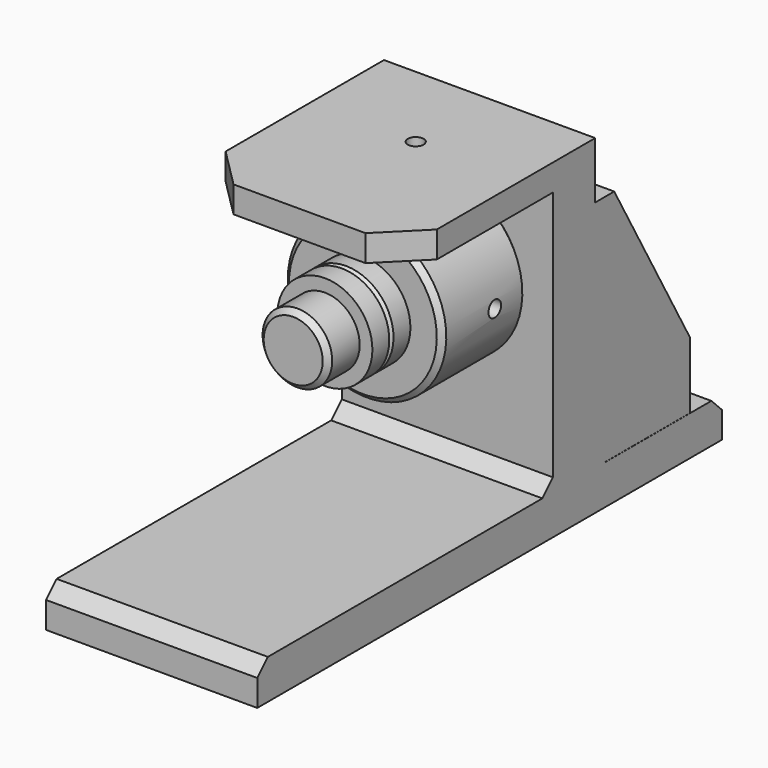
from build123d import *

# Parameters (mm, degrees)
F2_SIZE         = 2
F4_COPIES_COUNT = 4
F6_W            = 2
F6_H            = 10
F8_W            = 80
F8_H            = 90
F8_R            = 5
F9_DEPTH        = 10
F10_SIZE        = 15
F12_W           = 80
F12_H           = 100
F13_DEPTH       = 20
F15_DEPTH       = 80
F17_W           = 80
F17_H           = 15
F18_DEPTH       = 120
F18_DEPTH_BACK  = 100
F19_SIZE        = 5
F20_R           = 5
F21_DEPTH       = 10
F22_SIZE        = 2
F23_DEPTH       = 40
F23_DEPTH_BACK  = 40
F24_DEPTH       = 25
F24_DEPTH_BACK  = 25
F25_W           = 7
F25_H           = 20
F31_SIZE        = 2


# Not quite as in the source:
# - a pattern or mirror of a feature is missing from the dataset's text; its kind, count and spacing are read off the source's solid


with BuildPart() as f1:
    # F0 (on Right) → F1 (revolve)
    with BuildSketch(Plane.YZ):
        Polygon((-10, 18), (-10, 11), (40, 11), (40, 30), (0, 30), (0, 18), align=None)
    revolve(axis=Axis((0, 15, 0), (0, -1, 0)))

    # F2
    f2_edges = [f1.edges().sort_by_distance(p)[0] for p in [
        (0, -10, -18),
        (0, 0, -30),
        (0, 40, -30),
    ]]
    chamfer(f2_edges, length=F2_SIZE)

    # F3 (on Right) → F4 (revolve, cut)
    with BuildSketch(Plane.YZ):
        Polygon((22, 18), (25, 16.2679491924), (25, 30), (22, 30), align=None)
    f4 = revolve(axis=Axis((0, 25, 23.1339745962), (0, 0, 1)), mode=Mode.SUBTRACT)

    # F4_copies: F4 ×4 about axis
    f4_copies_axis = Axis((0, 0, 0), (0, 1, 0))
    for i in range(1, F4_COPIES_COUNT):
        add(f4.rotate(f4_copies_axis, i * 360 / F4_COPIES_COUNT), mode=Mode.SUBTRACT)


with BuildPart() as f7:
    # F6 (on Right) → F7 (revolve)
    with BuildSketch(Plane.YZ):
        with Locations((21, 41)):
            Rectangle(F6_W, F6_H)
    revolve(axis=Axis((0, 25, 40.9752885997), (0, 0, -1)))

    # F8 (on offset) → F9 (join)
    with BuildSketch(Plane.XY.offset(46)):
        with Locations((0, 15)):
            Rectangle(F8_W, F8_H)
        with Locations((0, 25)):
            Circle(F8_R, mode=Mode.SUBTRACT)
    extrude(amount=-F9_DEPTH)

    # F10
    f10_edges = [f7.edges().sort_by_distance(p)[0] for p in [
        (-40, -30, 41),
        (40, -30, 41),
    ]]
    chamfer(f10_edges, length=F10_SIZE)

    # F12 (on offset) → F13 (join)
    with BuildSketch(Plane.XZ.offset(-60)):
        with Locations((0, -14)):
            Rectangle(F12_W, F12_H)
    extrude(amount=F13_DEPTH)

    # F14 (on face) → F15 (join)
    with BuildSketch(Plane.YZ.offset(40)):
        Polygon((35, -64), (40, -64), (40, -59), align=None)
        Polygon((60, -59), (60, -64), (65, -64), align=None)
    extrude(amount=-F15_DEPTH)

    # F17 (on Front) → F18 (join, two sides)
    with BuildSketch(Plane.XZ) as f18_sk:
        with Locations((0, -71.5)):
            Rectangle(F17_W, F17_H)
    extrude(amount=-F18_DEPTH)
    extrude(f18_sk.sketch, amount=F18_DEPTH_BACK)

    # F19
    f19_edges = [f7.edges().sort_by_distance(p)[0] for p in [
        (0, 120, -64),
        (0, -100, -64),
    ]]
    chamfer(f19_edges, length=F19_SIZE)

    # F20 (on face) → F21 (join)
    with BuildSketch(Plane(origin=(0, 0, -79), x_dir=(1, 0, 0), z_dir=(0, 0, -1))):
        with Locations((0, 50)):
            Circle(F20_R)
        with Locations((0, -70)):
            Circle(F20_R)
    extrude(amount=F21_DEPTH)

    # F22
    f22_edges = [f7.edges().sort_by_distance(p)[0] for p in [
        (-5, -50, -89),
        (-5, 70, -89),
    ]]
    chamfer(f22_edges, length=F22_SIZE)

    # F16 (on Right) → F23 (join, two sides)
    with BuildSketch(Plane.YZ) as f23_sk:
        Polygon((69, 24.5257518999), (60, 24.5257518999), (60, -63.9528611181), (105, -63.9528611181), (105, -38.9528611181), align=None)
    extrude(amount=F23_DEPTH)
    extrude(f23_sk.sketch, amount=-F23_DEPTH_BACK)

    # F16 (on Right) → F24 (cut, two sides)
    with BuildSketch(Plane.YZ) as f24_sk:
        Polygon((69, 24.5257518999), (60, 24.5257518999), (60, -63.9528611181), (105, -63.9528611181), (105, -38.9528611181), align=None)
    extrude(amount=F24_DEPTH, mode=Mode.SUBTRACT)
    extrude(f24_sk.sketch, amount=-F24_DEPTH_BACK, mode=Mode.SUBTRACT)

    # F25 (on Right) → F26 (revolve, cut)
    with BuildSketch(Plane.YZ):
        with Locations((56.5, 10)):
            Rectangle(F25_W, F25_H)
    revolve(axis=Axis((0, 56.5, 0), (0, 1, 0)), mode=Mode.SUBTRACT)


with BuildPart() as f28_tool:
    # F27 (on Right) → F28 (revolve)
    with BuildSketch(Plane.YZ):
        Polygon((53, 13), (51, 15), (40, 15), (40, 14), (37, 14), (37, 15), (6, 15), (4, 13), (4, 0), (53, 0), align=None)
    revolve(axis=Axis((0, 28.5, 0), (0, 1, 0)))


with BuildPart() as f1_1:
    add(f1.part)

    # F28: cut by f28_tool
    add(f28_tool.part, mode=Mode.SUBTRACT)

    # F29 (on Right) → F30 (revolve)
    with BuildSketch(Plane.YZ):
        Polygon((-18, 18), (-18, 13.1793413311), (-33, 13.1793413311), (-33, 0), (-3, 0), (-3, 11), (-10, 11), (-10, 18), align=None)
    revolve(axis=Axis((0, -18, 0), (0, 1, 0)))

    # F31
    f31_edges = [f1_1.edges().sort_by_distance(p)[0] for p in [
        (0, -33, -13.179341),
    ]]
    chamfer(f31_edges, length=F31_SIZE)


with BuildPart() as f7_1:
    add(f7.part)

    # F28: cut by f28_tool
    add(f28_tool.part, mode=Mode.SUBTRACT)


solid = Compound([f1_1.part, f7_1.part])
